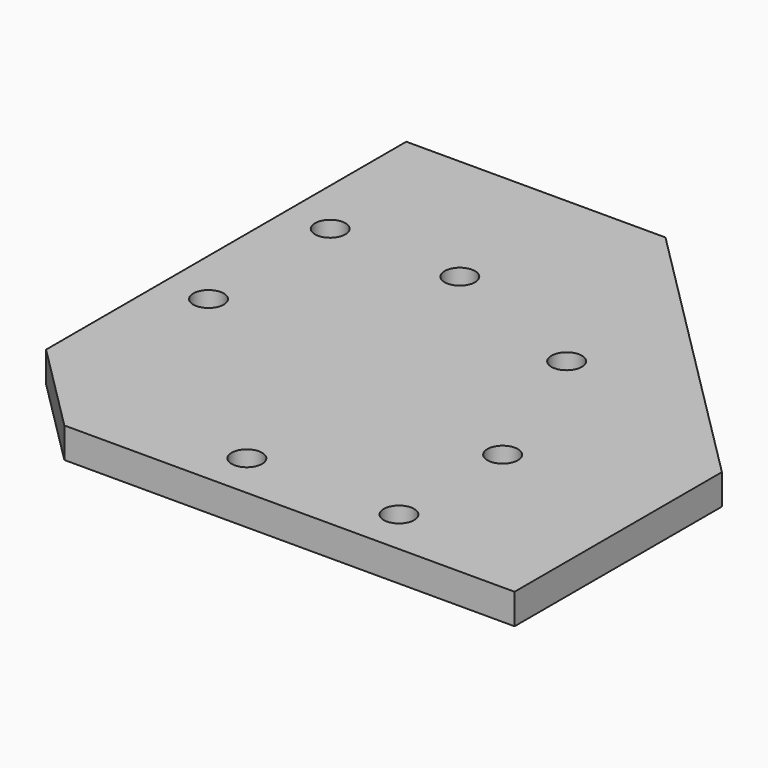
from build123d import *

# Parameters (mm, degrees)
F0_R     = 2.5
F1_DEPTH = 5


# Not quite as in the source:
# - a feature names something its author has since deleted; it is built from what else it names


with BuildPart() as f1:
    # F0 (on Top) → F1 (new body)
    with BuildSketch(Plane.XY):
        Polygon((-46.496636016, -24.5297024497), (-31.496636016, -39.5297024497), (42.503363984, -39.5297024497), (42.503363984, 3.0702975503), (-3.896636016, 49.4702975503), (-46.496636016, 49.4702975503), align=None)
        with Locations((-7.496636016, -32.0297024497)):
            Circle(F0_R, mode=Mode.SUBTRACT)
        with Locations((-38.996636016, -0.5297024497)):
            Circle(F0_R, mode=Mode.SUBTRACT)
        with Locations((17.503363984, -32.0297024497)):
            Circle(F0_R, mode=Mode.SUBTRACT)
        with Locations((17.503363984, -10.7297024497)):
            Circle(F0_R, mode=Mode.SUBTRACT)
        with Locations((-38.996636016, 24.4702975503)):
            Circle(F0_R, mode=Mode.SUBTRACT)
        with Locations((-17.696636016, 24.4702975503)):
            Circle(F0_R, mode=Mode.SUBTRACT)
        with Locations((7.703363984, 14.6702975503)):
            Circle(F0_R, mode=Mode.SUBTRACT)
    extrude(amount=F1_DEPTH)


solid = f1.part
